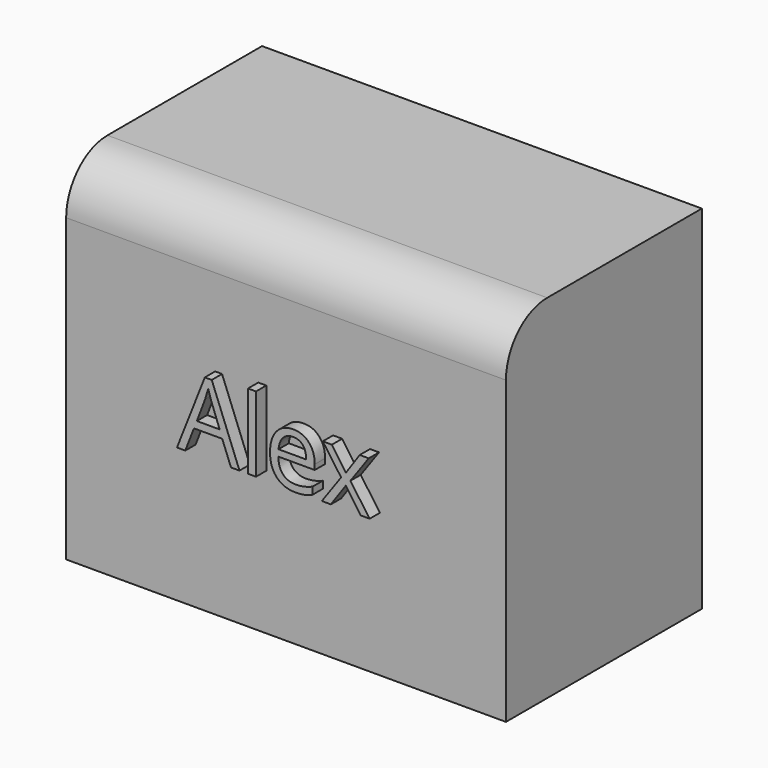
from build123d import *

# Parameters (mm, degrees)
F0_W         = 43.3427840471
F0_H         = 34.7322747111
F1_DEPTH     = 24.13
F2_T         = -2.54
F3_R         = 5.08
F4_TEXT_SIZE = 9.7371314445
F5_DEPTH     = 25.4


# Not quite as in the source:
# - Text() gives the source's letters only with a copy of the font that has no kerning and outlines rounded to 1/6400 em; it was checked with that copy


with BuildPart() as f1:
    # F0 (on Front) → F1 (new body)
    with BuildSketch(Plane.XZ):
        with Locations((0.0967476517, 17.3661373556)):
            Rectangle(F0_W, F0_H)
    extrude(amount=F1_DEPTH)

    # F2
    f2_openings = [f1.faces().sort_by_distance(p)[0] for p in [
        (0.096748, -12.065, 0),
    ]]
    offset(amount=F2_T, openings=f2_openings)

    # F3
    f3_edges = [f1.edges().sort_by_distance(p)[0] for p in [
        (0.096748, -24.13, 34.732275),
    ]]
    fillet(f3_edges, radius=F3_R)

    # F4 (on Front) → F5 (join)
    with BuildSketch(Plane.XZ):
        with Locations((-9.6397586167, 14.1091020778)):
            Text('Alex', F4_TEXT_SIZE, font='Open Sans', text_align=(TextAlign.LEFT, TextAlign.BOTTOM))
    extrude(amount=F5_DEPTH)


solid = f1.part
